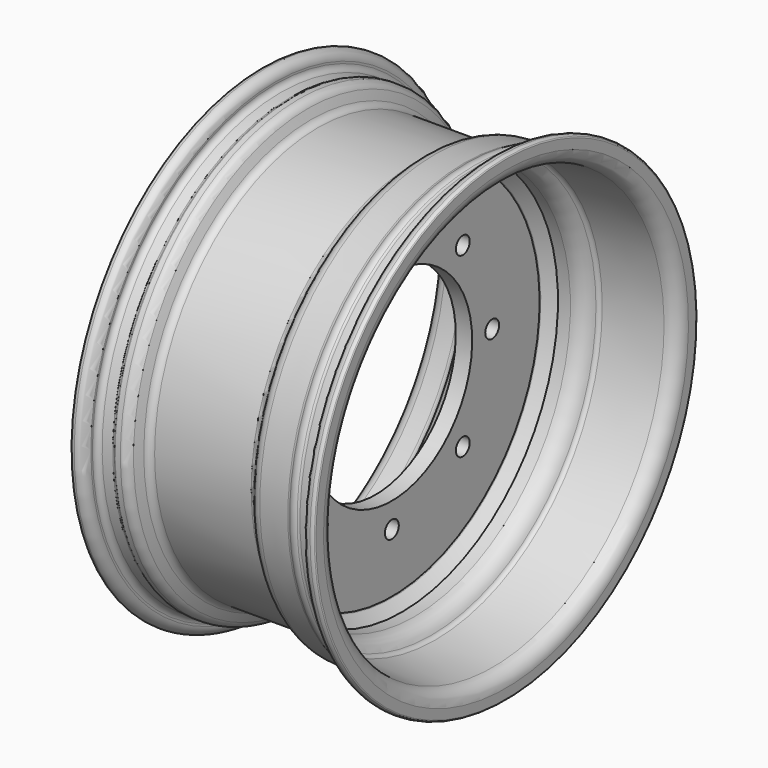
from build123d import *

# Parameters (mm, degrees)
F2_SCALE        = 2
F4_D            = 19
F4_COPIES_COUNT = 8


# Not quite as in the source:
# - ends of sketch curves that miss each other by under 0.0002 mm in the source are joined
# - a pattern or mirror of a feature is missing from the dataset's text; its kind, count and spacing are read off the source's solid


with BuildPart() as f1:
    # F0 (on Front) → F1 (revolve)
    with BuildSketch(Plane.XZ):
        with BuildLine():
            Line((-59.3774947068, 125.3587021862), (-59.3774947068, 126.4546972823))
            ThreePointArc((-59.3774947068, 126.4546972823), (-60.8588365516, 130.03094887), (-64.4350881393, 131.5122907147))
            ThreePointArc((-64.4350881393, 131.5122907147), (-65.4343638443, 131.3591542469), (-66.3419257453, 130.9138070696))
            ThreePointArc((-66.3419257453, 130.9138070696), (-66.5882719889, 130.63401554), (-66.6771172223, 130.2719706726))
            Line((-66.6771172223, 130.2719706726), (-66.6771172223, 125.0633919127))
            ThreePointArc((-66.6771172223, 125.0633919127), (-66.482618085, 123.3300296057), (-65.9087927875, 121.682880757))
            ThreePointArc((-65.9087927875, 121.682880757), (-63.307914247, 118.6330200999), (-59.5377401385, 117.2721356805))
            Line((-59.5377401385, 117.2721356805), (-49.5930421254, 116.4020858831))
            ThreePointArc((-49.5930421254, 116.4020858831), (-46.5853470395, 115.2625721401), (-44.6162629101, 112.7194580906))
            ThreePointArc((-44.6162629101, 112.7194580906), (-41.1625787231, 108.4545206728), (-35.9144230058, 106.85))
            Line((-35.9144230058, 106.85), (-9.7140138479, 106.85))
            Line((-9.7140138479, 106.85), (-4.5, 106.85))
            Line((-4.5, 106.85), (4.5, 106.85))
            Line((4.5, 106.85), (10.0992387742, 106.85))
            Line((10.0992387742, 106.85), (16.9436956085, 106.85))
            ThreePointArc((16.9436956085, 106.85), (22.4251553149, 108.5046629344), (26.0755268905, 112.9159096174))
            ThreePointArc((26.0755268905, 112.9159096174), (26.9427979858, 114.0117789594), (28.2514212765, 114.5022829559))
            Line((28.2514212765, 114.5022829559), (59.9229640063, 117.2731849198))
            ThreePointArc((59.9229640063, 117.2731849198), (65.0075805706, 119.7806360461), (67.0623421486, 125.0644409723))
            Line((67.0623421486, 125.0644409723), (67.0623411058, 130.2719706726))
            ThreePointArc((67.0623411058, 130.2719706726), (66.9734967171, 130.6340159193), (66.7271505795, 130.9138084349))
            ThreePointArc((66.7271505795, 130.9138084349), (65.8195878649, 131.3591545311), (64.8203120228, 131.5122907148))
            ThreePointArc((64.8203120228, 131.5122907148), (61.2440604351, 130.03094887), (59.7627185904, 126.4546972823))
            Line((59.7627185904, 126.4546972823), (59.7627185903, 125.3597512458))
            ThreePointArc((59.7627185903, 125.3597512458), (58.9408175176, 123.2462281069), (56.9069708435, 122.2432479785))
            Line((56.9069708435, 122.2432479785), (51.5454233807, 121.7741729888))
            ThreePointArc((51.5454233807, 121.7741729888), (50.8159764062, 121.7957947298), (50.1113861259, 121.9858287981))
            ThreePointArc((50.1113861259, 121.9858287981), (47.8647261886, 122.3174224608), (45.70977758, 121.6007415585))
            ThreePointArc((45.70977758, 121.6007415585), (45.0488899564, 121.2912445121), (44.3342795748, 121.1432822635))
            Line((44.3342795748, 121.1432822635), (27.863538289, 119.7022761349))
            ThreePointArc((27.863538289, 119.7022761349), (23.9360777257, 118.2296017987), (21.334324273, 114.9395266697))
            ThreePointArc((21.334324273, 114.9395266697), (19.6052745797, 112.8484561771), (17.00780608, 112.0640159336))
            Line((17.00780608, 112.0640159336), (-35.9144344767, 112.0640159335))
            ThreePointArc((-35.9144344767, 112.0640159335), (-38.2469432811, 112.7771380477), (-39.7819144418, 114.6726601416))
            Line((-39.7819144418, 114.6726601416), (-41.6632173981, 119.3290611948))
            ThreePointArc((-41.6632173981, 119.3290611948), (-43.5243685327, 121.6273844601), (-46.3525377329, 122.4920415438))
            Line((-46.3525377329, 122.4920415438), (-49.2101697889, 122.4920415438))
            ThreePointArc((-49.2101697889, 122.4920415438), (-49.5195674906, 122.4282391081), (-49.7784889992, 122.2472488486))
            ThreePointArc((-49.7784889992, 122.2472488486), (-50.3595799373, 121.8596366017), (-51.0514529348, 121.7636058247))
            Line((-51.0514529348, 121.7636058247), (-56.5217459526, 122.2421985139))
            ThreePointArc((-56.5217459526, 122.2421985139), (-58.5555925913, 123.2451790473), (-59.3774947068, 125.3587021862))
        make_face()
        Polygon((-4.5, 106.85), (-9.7140138479, 106.85), (-4.5, 101.6359882377), align=None)
        Polygon((-4.5, 106.85), (-4.5, 101.6359882377), (-4.5, 55.05), (4.5, 55.05), (4.5, 101.2507633114), (4.5, 106.85), align=None)
        Polygon((10.0992387742, 106.85), (4.5, 106.85), (4.5, 101.2507633114), (4.8852249263, 101.6359882377), align=None)
    revolve(axis=Axis((0, 0, 0), (1, 0, 0)))


with BuildPart() as f1_1:
    # F2: moved
    add(f1.part.scale(F2_SCALE))

    # F4 (through all)
    with Locations(Plane(origin=(-9, 0, 0), x_dir=(0, -1, 0), z_dir=(-1, 0, 0))):
        with Locations((0, 137.5)):
            f4 = Hole(F4_D / 2)

    # F4_copies: F4 ×8 about axis
    f4_copies_axis = Axis((0, 0, 0), (1, 0, 0))
    for i in range(1, F4_COPIES_COUNT):
        add(f4.rotate(f4_copies_axis, i * 360 / F4_COPIES_COUNT), mode=Mode.SUBTRACT)


solid = f1_1.part
